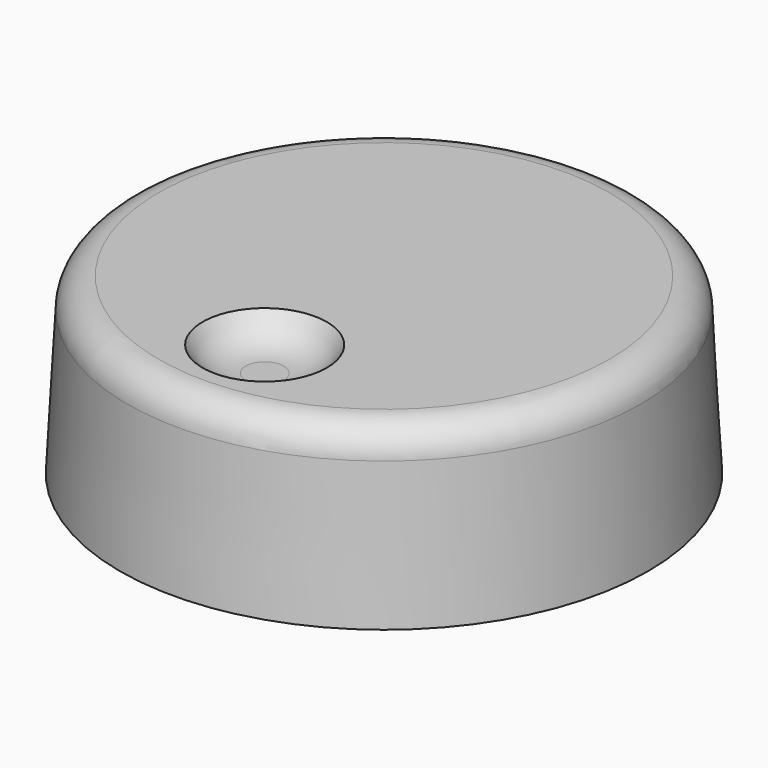
from build123d import *

# Parameters (mm, degrees)
F0_R      = 26.9875
F1_DEPTH  = 17.78
F1_TAPER  = 3
F2_R      = 3.175
F3_R      = 6.35
F4_DEPTH  = 2.54
F7_DEPTH  = 12.7
F8_R      = 5.08
F9_R      = 2.54
F11_DEPTH = 15.24


# Not quite as in the source:
# - a fillet or chamfer that OpenCascade refuses, or shapes differently, is made with other operations: its cross-section is extruded or revolved along the edge and cut away or added


with BuildPart() as f1:
    # F0 (on Top) → F1 (new body)
    with BuildSketch(Plane.XY):
        Circle(F0_R)
    extrude(amount=F1_DEPTH, taper=F1_TAPER)

    # F2
    f2_edges = [f1.edges().sort_by_distance(p)[0] for p in [
        (-26.05569, 0, 17.78),
    ]]
    fillet(f2_edges, radius=F2_R)

    # F3 (on face) → F4 (cut)
    with BuildSketch(Plane.XY.offset(17.78)):
        with Locations((0, -15.24)):
            Circle(F3_R)
    extrude(amount=-F4_DEPTH, mode=Mode.SUBTRACT)

    # F5: fillet of radius 5.08 on 1 edges, made by hand

    # F5_s1 → F5_t2 (revolve)
    with BuildSketch(Plane.XZ.offset(15.24)):
        with BuildLine():
            ThreePointArc((6.35, 17.78), (4.4905909488, 15.9205909488), (1.9505909488, 15.24))
            Line((1.9505909488, 15.24), (6.35, 15.24))
            Line((6.35, 15.24), (6.35, 17.78))
        make_face()
    revolve(axis=Axis((0, -15.24, 15.24), (0, 0, 1)))

    # F6 (on face) → F7 (cut)
    with BuildSketch(Plane(origin=(0, 0, 0), x_dir=(1, 0, 0), z_dir=(0, 0, -1))):
        with BuildLine():
            ThreePointArc((1.27, 9.4399536545), (0, -9.525), (-1.27, 9.4399536545))
            Line((-1.27, 9.4399536545), (-1.27, 23.7786092161))
            ThreePointArc((-1.27, 23.7786092161), (0, -23.8125), (1.27, 23.7786092161))
            Line((1.27, 23.7786092161), (1.27, 9.4399536545))
        make_face()
    extrude(amount=-F7_DEPTH, mode=Mode.SUBTRACT)

    # F8
    f8_edges = [f1.edges().sort_by_distance(p)[0] for p in [
        (0, 23.8125, 12.7),
    ]]
    fillet(f8_edges, radius=F8_R)

    # F9
    f9_edges = [f1.edges().sort_by_distance(p)[0] for p in [
        (0, 9.525, 12.7),
    ]]
    fillet(f9_edges, radius=F9_R)

    # F10 (on face) → F11 (cut)
    with BuildSketch(Plane(origin=(0, 0, 0), x_dir=(1, 0, 0), z_dir=(0, 0, -1))):
        with BuildLine():
            Line((-2.6396454307, -1.524), (2.6396454307, -1.524))
            ThreePointArc((2.6396454307, -1.524), (0, 3.048), (-2.6396454307, -1.524))
        make_face()
    extrude(amount=-F11_DEPTH, mode=Mode.SUBTRACT)


solid = f1.part
